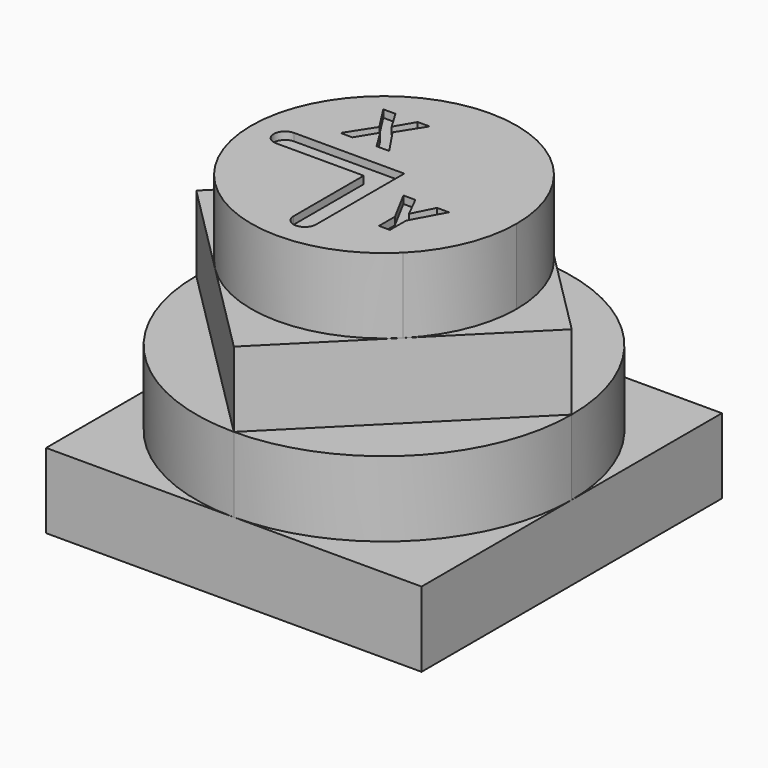
from build123d import *

# Parameters (mm, degrees)
F1_DEPTH     = 10
F2_DEPTH     = 20
F3_DEPTH     = 30
F4_DEPTH     = 40
F5_TEXT_SIZE = 9.7222222222
F6_DEPTH     = 1


# Not quite as in the source:
# - a feature names something its author has since deleted; it is built from what else it names
# - Text() gives the source's letters only with a copy of the font that has no kerning and outlines rounded to 1/6400 em; it was checked with that copy


with BuildPart() as f1:
    # F0 (on Top) → F1 (new body)
    with BuildSketch(Plane.XY):
        with BuildLine():
            Line((25, 0), (25, 25))
            Line((25, 25), (0, 25))
            ThreePointArc((0, 25), (17.6776695297, 17.6776695297), (25, 0))
        make_face()
        with BuildLine():
            ThreePointArc((-25, 0), (-17.6776695297, 17.6776695297), (0, 25))
            Line((0, 25), (-25, 25))
            Line((-25, 25), (-25, 0))
        make_face()
        with BuildLine():
            Line((-12.4999999822, 12.5000000178), (0, 25))
            ThreePointArc((0, 25), (-17.6776695297, 17.6776695297), (-25, 0))
            Line((-25, 0), (-12.4999999822, 12.5000000178))
        make_face()
        with BuildLine():
            Line((12.4999999904, 12.5000000096), (0, 25))
            Line((0, 25), (-12.4999999822, 12.5000000178))
            ThreePointArc((-12.4999999822, 12.5000000178), (5.8e-09, 17.6776695297), (12.4999999904, 12.5000000096))
        make_face()
        with BuildLine():
            ThreePointArc((25, 0), (17.6776695297, 17.6776695297), (0, 25))
            Line((0, 25), (12.4999999904, 12.5000000096))
            Line((12.4999999904, 12.5000000096), (25, 0))
        make_face()
        with BuildLine():
            Line((25, -25), (25, 0))
            ThreePointArc((25, 0), (17.6776695297, -17.6776695297), (0, -25))
            Line((0, -25), (25, -25))
        make_face()
        with BuildLine():
            Line((12.500000015, -12.499999985), (25, 0))
            Line((25, 0), (12.4999999904, 12.5000000096))
            ThreePointArc((12.4999999904, 12.5000000096), (16.3320370584, 6.7649512581), (17.6776695297, 0))
            ThreePointArc((17.6776695297, 0), (16.332037065, -6.764951242), (12.500000015, -12.499999985))
        make_face()
        with BuildLine():
            ThreePointArc((0, -25), (17.6776695297, -17.6776695297), (25, 0))
            Line((25, 0), (12.500000015, -12.499999985))
            Line((12.500000015, -12.499999985), (0, -25))
        make_face()
        with BuildLine():
            ThreePointArc((0, -25), (-17.6776695297, -17.6776695297), (-25, 0))
            Line((-25, 0), (-25, -25))
            Line((-25, -25), (0, -25))
        make_face()
        with BuildLine():
            Line((-12.4999999402, -12.5000000598), (-25, 0))
            ThreePointArc((-25, 0), (-17.6776695297, -17.6776695297), (0, -25))
            Line((0, -25), (-12.4999999402, -12.5000000598))
        make_face()
        with BuildLine():
            Line((-12.4999999822, 12.5000000178), (-25, 0))
            Line((-25, 0), (-12.4999999402, -12.5000000598))
            ThreePointArc((-12.4999999402, -12.5000000598), (-17.6776695297, -2.96e-08), (-12.4999999822, 12.5000000178))
        make_face()
        with BuildLine():
            Line((-12.4999999402, -12.5000000598), (0, -25))
            Line((0, -25), (12.500000015, -12.499999985))
            ThreePointArc((12.500000015, -12.499999985), (5.28e-08, -17.6776695297), (-12.4999999402, -12.5000000598))
        make_face()
        with BuildLine():
            ThreePointArc((12.4999999904, 12.5000000096), (5.8e-09, 17.6776695297), (-12.4999999822, 12.5000000178))
            ThreePointArc((-12.4999999822, 12.5000000178), (-17.6776695297, -2.96e-08), (-12.4999999402, -12.5000000598))
            ThreePointArc((-12.4999999402, -12.5000000598), (5.28e-08, -17.6776695297), (12.500000015, -12.499999985))
            ThreePointArc((12.500000015, -12.499999985), (16.332037065, -6.764951242), (17.6776695297, 0))
            ThreePointArc((17.6776695297, 0), (16.3320370584, 6.7649512581), (12.4999999904, 12.5000000096))
        make_face()
    extrude(amount=F1_DEPTH)

    # F0 (on Top) → F2 (join)
    with BuildSketch(Plane.XY):
        with BuildLine():
            Line((-12.4999999402, -12.5000000598), (-25, 0))
            ThreePointArc((-25, 0), (-17.6776695297, -17.6776695297), (0, -25))
            Line((0, -25), (-12.4999999402, -12.5000000598))
        make_face()
        with BuildLine():
            Line((-12.4999999822, 12.5000000178), (0, 25))
            ThreePointArc((0, 25), (-17.6776695297, 17.6776695297), (-25, 0))
            Line((-25, 0), (-12.4999999822, 12.5000000178))
        make_face()
        with BuildLine():
            ThreePointArc((12.4999999904, 12.5000000096), (5.8e-09, 17.6776695297), (-12.4999999822, 12.5000000178))
            ThreePointArc((-12.4999999822, 12.5000000178), (-17.6776695297, -2.96e-08), (-12.4999999402, -12.5000000598))
            ThreePointArc((-12.4999999402, -12.5000000598), (5.28e-08, -17.6776695297), (12.500000015, -12.499999985))
            ThreePointArc((12.500000015, -12.499999985), (16.332037065, -6.764951242), (17.6776695297, 0))
            ThreePointArc((17.6776695297, 0), (16.3320370584, 6.7649512581), (12.4999999904, 12.5000000096))
        make_face()
        with BuildLine():
            ThreePointArc((25, 0), (17.6776695297, 17.6776695297), (0, 25))
            Line((0, 25), (12.4999999904, 12.5000000096))
            Line((12.4999999904, 12.5000000096), (25, 0))
        make_face()
        with BuildLine():
            ThreePointArc((0, -25), (17.6776695297, -17.6776695297), (25, 0))
            Line((25, 0), (12.500000015, -12.499999985))
            Line((12.500000015, -12.499999985), (0, -25))
        make_face()
        with BuildLine():
            Line((12.500000015, -12.499999985), (25, 0))
            Line((25, 0), (12.4999999904, 12.5000000096))
            ThreePointArc((12.4999999904, 12.5000000096), (16.3320370584, 6.7649512581), (17.6776695297, 0))
            ThreePointArc((17.6776695297, 0), (16.332037065, -6.764951242), (12.500000015, -12.499999985))
        make_face()
        with BuildLine():
            Line((-12.4999999402, -12.5000000598), (0, -25))
            Line((0, -25), (12.500000015, -12.499999985))
            ThreePointArc((12.500000015, -12.499999985), (5.28e-08, -17.6776695297), (-12.4999999402, -12.5000000598))
        make_face()
        with BuildLine():
            Line((-12.4999999822, 12.5000000178), (-25, 0))
            Line((-25, 0), (-12.4999999402, -12.5000000598))
            ThreePointArc((-12.4999999402, -12.5000000598), (-17.6776695297, -2.96e-08), (-12.4999999822, 12.5000000178))
        make_face()
        with BuildLine():
            Line((12.4999999904, 12.5000000096), (0, 25))
            Line((0, 25), (-12.4999999822, 12.5000000178))
            ThreePointArc((-12.4999999822, 12.5000000178), (5.8e-09, 17.6776695297), (12.4999999904, 12.5000000096))
        make_face()
    extrude(amount=F2_DEPTH)

    # F0 (on Top) → F3 (join)
    with BuildSketch(Plane.XY):
        with BuildLine():
            Line((-12.4999999402, -12.5000000598), (0, -25))
            Line((0, -25), (12.500000015, -12.499999985))
            ThreePointArc((12.500000015, -12.499999985), (5.28e-08, -17.6776695297), (-12.4999999402, -12.5000000598))
        make_face()
        with BuildLine():
            Line((12.500000015, -12.499999985), (25, 0))
            Line((25, 0), (12.4999999904, 12.5000000096))
            ThreePointArc((12.4999999904, 12.5000000096), (16.3320370584, 6.7649512581), (17.6776695297, 0))
            ThreePointArc((17.6776695297, 0), (16.332037065, -6.764951242), (12.500000015, -12.499999985))
        make_face()
        with BuildLine():
            ThreePointArc((12.4999999904, 12.5000000096), (5.8e-09, 17.6776695297), (-12.4999999822, 12.5000000178))
            ThreePointArc((-12.4999999822, 12.5000000178), (-17.6776695297, -2.96e-08), (-12.4999999402, -12.5000000598))
            ThreePointArc((-12.4999999402, -12.5000000598), (5.28e-08, -17.6776695297), (12.500000015, -12.499999985))
            ThreePointArc((12.500000015, -12.499999985), (16.332037065, -6.764951242), (17.6776695297, 0))
            ThreePointArc((17.6776695297, 0), (16.3320370584, 6.7649512581), (12.4999999904, 12.5000000096))
        make_face()
        with BuildLine():
            Line((12.4999999904, 12.5000000096), (0, 25))
            Line((0, 25), (-12.4999999822, 12.5000000178))
            ThreePointArc((-12.4999999822, 12.5000000178), (5.8e-09, 17.6776695297), (12.4999999904, 12.5000000096))
        make_face()
        with BuildLine():
            Line((-12.4999999822, 12.5000000178), (-25, 0))
            Line((-25, 0), (-12.4999999402, -12.5000000598))
            ThreePointArc((-12.4999999402, -12.5000000598), (-17.6776695297, -2.96e-08), (-12.4999999822, 12.5000000178))
        make_face()
    extrude(amount=F3_DEPTH)

    # F0 (on Top) → F4 (join)
    with BuildSketch(Plane.XY):
        with BuildLine():
            ThreePointArc((12.4999999904, 12.5000000096), (5.8e-09, 17.6776695297), (-12.4999999822, 12.5000000178))
            ThreePointArc((-12.4999999822, 12.5000000178), (-17.6776695297, -2.96e-08), (-12.4999999402, -12.5000000598))
            ThreePointArc((-12.4999999402, -12.5000000598), (5.28e-08, -17.6776695297), (12.500000015, -12.499999985))
            ThreePointArc((12.500000015, -12.499999985), (16.332037065, -6.764951242), (17.6776695297, 0))
            ThreePointArc((17.6776695297, 0), (16.3320370584, 6.7649512581), (12.4999999904, 12.5000000096))
        make_face()
    extrude(amount=F4_DEPTH)

    # F5 (on face) → F6 (cut)
    with BuildSketch(Plane.XY.offset(40)):
        with BuildLine():
            ThreePointArc((-1.5, -13.1776695297), (0, -14.6776695297), (1.5, -13.1776695297))
            Line((1.5, -13.1776695297), (1.5, 1.5))
            Line((1.5, 1.5), (-13.1776695297, 1.5))
            ThreePointArc((-13.1776695297, 1.5), (-14.6776695297, 0), (-13.1776695297, -1.5))
            Line((-13.1776695297, -1.5), (-1.5, -1.5))
            Line((-1.5, -1.5), (-1.5, -13.1776695297))
        make_face()
        with Locations((4.5, -9.3388347648)):
            Text('Y', F5_TEXT_SIZE, font='Open Sans', font_style=FontStyle.BOLD, text_align=(TextAlign.LEFT, TextAlign.BOTTOM))
        with Locations((-9.3965604593, 4.5)):
            Text('X', F5_TEXT_SIZE, font='Open Sans', font_style=FontStyle.BOLD, text_align=(TextAlign.LEFT, TextAlign.BOTTOM))
    extrude(amount=-F6_DEPTH, mode=Mode.SUBTRACT)


solid = f1.part
